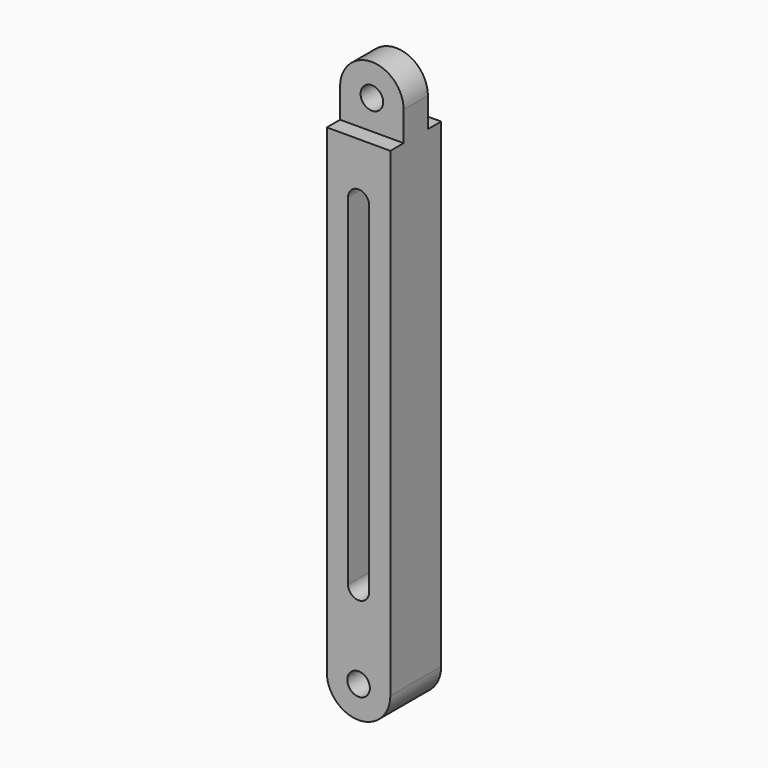
from build123d import *

# Parameters (mm, degrees)
F0_W     = 5.588
F0_H     = 33.6042
F0_R     = 0.9906
F2_DEPTH = 5.588
F3_W     = 1.4605
F3_H     = 2.5908
F3_H_2   = 2.794
F4_DEPTH = 5.589


# Not quite as in the source:
# - the program builds the solid bodies; features that only make, move or delete a surface that nothing else refers to are left out


with BuildPart() as f2:
    # F0 (on Front) → F2 (new body)
    with BuildSketch(Plane.XZ):
        Rectangle(F0_W, F0_H)
        with BuildLine():
            ThreePointArc((-0.9271, 14.986), (0, 15.9131), (0.9271, 14.986))
            Line((0.9271, 14.986), (0.9271, -14.986))
            ThreePointArc((0.9271, -14.986), (0, -15.9131), (-0.9271, -14.986))
            Line((-0.9271, -14.986), (-0.9271, 14.986))
        make_face(mode=Mode.SUBTRACT)
        with BuildLine():
            Line((-2.794, 16.8021), (2.794, 16.8021))
            Line((2.794, 16.8021), (2.794, 22.3901))
            ThreePointArc((2.794, 22.3901), (0, 25.1841), (-2.794, 22.3901))
            Line((-2.794, 22.3901), (-2.794, 16.8021))
        make_face()
        with Locations((0, 22.3901)):
            Circle(F0_R, mode=Mode.SUBTRACT)
        with BuildLine():
            Line((2.794, -22.3901), (2.794, -16.8021))
            Line((2.794, -16.8021), (-2.794, -16.8021))
            Line((-2.794, -16.8021), (-2.794, -22.3901))
            ThreePointArc((-2.794, -22.3901), (0, -25.1841), (2.794, -22.3901))
        make_face()
        with Locations((0, -22.3901)):
            Circle(F0_R, mode=Mode.SUBTRACT)
    extrude(amount=F2_DEPTH)

    # F3 (on face) → F4 (cut, through all)
    with BuildSketch(Plane(origin=(-2.794, 0, 0), x_dir=(0, -1, 0), z_dir=(-1, 0, 0))):
        with Locations((0.73025, 21.0947)):
            Rectangle(F3_W, F3_H)
        with Locations((0.73025, 23.7871)):
            Rectangle(F3_W, F3_H_2)
        with Locations((4.85775, 23.7871)):
            Rectangle(F3_W, F3_H_2)
        with Locations((4.85775, 21.0947)):
            Rectangle(F3_W, F3_H)
    extrude(amount=-F4_DEPTH, mode=Mode.SUBTRACT)


solid = f2.part
